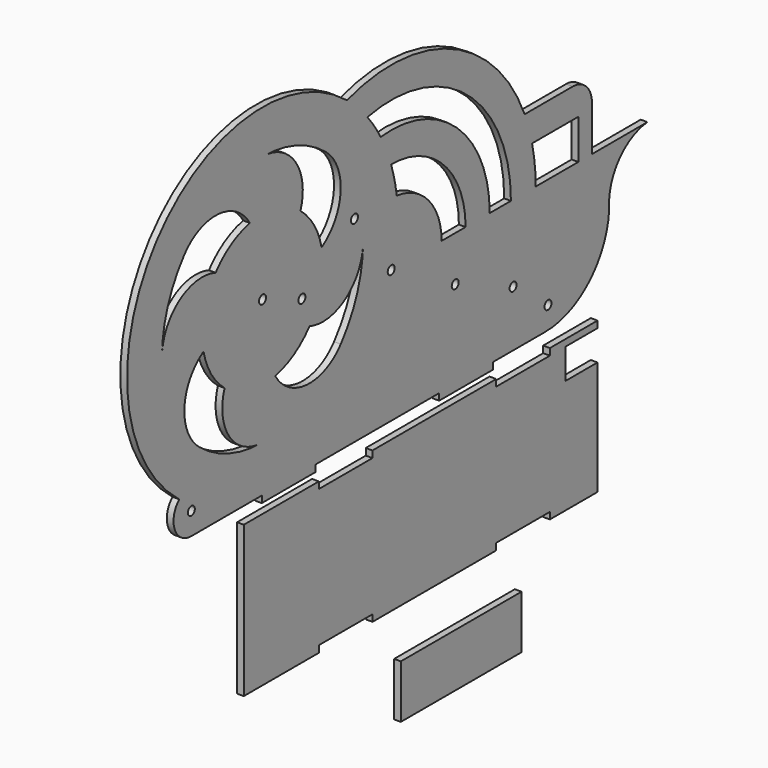
from build123d import *

# Parameters (mm, degrees)
F0_R     = 1.651
F0_W     = 25.4
F0_H     = 2.54
F1_DEPTH = 2.54
F3_DEPTH = 2.54
F2_W     = 57.15
F2_H     = 20.1916538


# Not quite as in the source:
# - a feature names something its author has since deleted; it is built from what else it names


with BuildPart() as f1:
    # F0 (on Right) → F1 (new body)
    with BuildSketch(Plane.YZ):
        with BuildLine():
            Line((-110.3395098078, -68.216781003), (-77.0102134189, -68.216781003))
            Line((-77.0102134189, -68.216781003), (-51.6102134189, -68.216781003))
            Line((-51.6102134189, -68.216781003), (6.9758426398, -68.216781003))
            Line((6.9758426398, -68.216781003), (32.3758426398, -68.216781003))
            Line((32.3758426398, -68.216781003), (57.100551478, -68.216781003))
            ThreePointArc((57.100551478, -68.216781003), (79.1760571871, -58.7450905637), (87.4551682283, -36.1952082478))
            ThreePointArc((87.4551682283, -36.1952082478), (93.1827609105, -23.7752479136), (105.5495773538, -17.933794011))
            Line((105.5495773538, -17.933794011), (79.3032324412, -17.933794011))
            Line((79.3032324412, -17.933794011), (79.3032324412, -0.7903648026))
            ThreePointArc((79.3032324412, -0.7903648026), (76.6409185109, 5.6370295953), (70.2135241129, 8.2993435257))
            Line((70.2135241129, 8.2993435257), (47.4198818769, 8.2993435257))
            ThreePointArc((47.4198818769, 8.2993435257), (12.9543250307, 44.1398405436), (-36.6774012974, 47.1577167678))
            ThreePointArc((-36.6774012974, 47.1577167678), (-127.0218705021, 36.6937065388), (-116.0831372229, -53.5945138457))
            ThreePointArc((-116.0831372229, -53.5945138457), (-118.1944438098, -62.8630173745), (-110.3395098078, -68.216781003))
        make_face()
        with Locations((-110.3395098078, -59.7775988281)):
            Circle(F0_R, mode=Mode.SUBTRACT)
        with BuildLine():
            ThreePointArc((-106.5792463676, -40.0513765479), (-113.6163335987, -24.0126518115), (-104.5836338962, -9.0069321035))
            ThreePointArc((-104.5836338962, -9.0069321035), (-100.986725964, -17.9768034164), (-94.6055715395, -25.2347098813))
            ThreePointArc((-94.6055715395, -25.2347098813), (-92.199319164, -42.5832325093), (-76.6450592973, -50.6347098813))
            ThreePointArc((-76.6450592973, -50.6347098813), (-92.5200592973, -47.9109904866), (-106.5792463676, -40.0513765479))
        make_face(mode=Mode.SUBTRACT)
        with BuildLine():
            ThreePointArc((-70.6478370751, -30.9482844801), (-61.6779657622, -27.3513765479), (-54.4200592973, -20.9702221234))
            ThreePointArc((-54.4200592973, -20.9702221234), (-37.0715366693, -18.5639697479), (-29.0200592973, -3.0097098813))
            ThreePointArc((-29.0200592973, -3.0097098813), (-31.743778692, -18.8847098813), (-39.6033926307, -32.9438969515))
            ThreePointArc((-39.6033926307, -32.9438969515), (-55.6421173671, -39.9809841827), (-70.6478370751, -30.9482844801))
        make_face(mode=Mode.SUBTRACT)
        with Locations((-57.9914643632, -10.3356258236)):
            Circle(F0_R, mode=Mode.SUBTRACT)
        with Locations((41.94092891, -46.9549127524)):
            Circle(F0_R, mode=Mode.SUBTRACT)
        with Locations((58.4825998644, -59.7775988281)):
            Circle(F0_R, mode=Mode.SUBTRACT)
        with Locations((14.561701, -35.0126066428)):
            Circle(F0_R, mode=Mode.SUBTRACT)
        with Locations((-15.7277009394, -17.933794011)):
            Circle(F0_R, mode=Mode.SUBTRACT)
        with BuildLine():
            Line((72.8437239482, -17.933794011), (52.6520820419, -17.933794011))
            ThreePointArc((52.6520820419, -17.933794011), (52.2295051274, -10.343480173), (50.9669973093, -2.8469803618))
            Line((50.9669973093, -2.8469803618), (72.8437239482, -2.8469803618))
            Line((72.8437239482, -2.8469803618), (72.8437239482, -17.933794011))
        make_face(mode=Mode.SUBTRACT)
        with BuildLine():
            ThreePointArc((-124.2700592973, -3.0097098813), (-121.5463399027, 12.8652901187), (-113.686725964, 26.924477189))
            ThreePointArc((-113.686725964, 26.924477189), (-97.6480012275, 33.9615644202), (-82.6422815195, 24.9288647176))
            ThreePointArc((-82.6422815195, 24.9288647176), (-91.6121528324, 21.3319567854), (-98.8700592973, 14.9508023609))
            ThreePointArc((-98.8700592973, 14.9508023609), (-116.2185819254, 12.5445499854), (-124.2700592973, -3.0097098813))
        make_face(mode=Mode.SUBTRACT)
        with Locations((-76.6450592973, -3.0097098813)):
            Circle(F0_R, mode=Mode.SUBTRACT)
        with Locations((-33.1285902436, 6.2196841001)):
            Circle(F0_R, mode=Mode.SUBTRACT)
        with BuildLine():
            ThreePointArc((-46.7108722271, 34.0319567854), (-39.6737849959, 17.993232049), (-48.7064846984, 2.987512341))
            ThreePointArc((-48.7064846984, 2.987512341), (-52.3033926307, 11.9573836539), (-58.6845470552, 19.2152901187))
            ThreePointArc((-58.6845470552, 19.2152901187), (-61.0907994306, 36.5638127468), (-76.6450592973, 44.6152901187))
            ThreePointArc((-76.6450592973, 44.6152901187), (-60.7700592973, 41.8915707241), (-46.7108722271, 34.0319567854))
        make_face(mode=Mode.SUBTRACT)
        with BuildLine():
            ThreePointArc((8.1256330932, -17.933794011), (2.0413714041, -2.0202270784), (-13.1075925996, 5.7752037906))
            ThreePointArc((-13.1075925996, 5.7752037906), (-14.1849392561, 11.581992796), (-15.7918139924, 17.2650754062))
            ThreePointArc((-15.7918139924, 17.2650754062), (9.1390218846, 6.9782636063), (19.4712268672, -17.933794011))
            Line((19.4712268672, -17.933794011), (8.1256330932, -17.933794011))
        make_face(mode=Mode.SUBTRACT)
        with BuildLine():
            ThreePointArc((-26.9908731892, 37.5938144058), (20.1332877639, 25.9314979047), (40.9306995465, -17.933794011))
            Line((40.9306995465, -17.933794011), (30.8992126275, -17.933794011))
            ThreePointArc((30.8992126275, -17.933794011), (15.4225371964, 16.7610432542), (-20.7332734529, 28.4236575215))
            ThreePointArc((-20.7332734529, 28.4236575215), (-23.6633025042, 33.1443746694), (-26.9908731892, 37.5938144058))
        make_face(mode=Mode.SUBTRACT)
        with Locations((-64.3102134189, -69.486781003)):
            Rectangle(F0_W, F0_H)
        with Locations((19.6758426398, -69.486781003)):
            Rectangle(F0_W, F0_H)
    extrude(amount=F1_DEPTH)


with BuildPart() as f3:
    # F2 (on Right) → F3 (new body)
    with BuildSketch(Plane.YZ):
        Polygon((-50.0091612339, -74.4957265361), (-85.5189124058, -74.4957265361), (-85.5189124058, -131.6457265361), (-50.0091612339, -131.6457265361), (-50.0091612339, -129.1057265361), (-24.6091612339, -129.1057265361), (-24.6091612339, -131.6457265361), (33.9769039661, -131.6457265361), (33.9769039661, -129.1057265361), (59.3769039661, -129.1057265361), (59.3769039661, -131.6457265361), (81.9211387942, -131.6457265361), (81.9211387942, -88.4657265361), (66.6811387942, -88.4657265361), (66.6811387942, -77.0357265361), (81.9211387942, -77.0357265361), (81.9211387942, -74.4957265361), (59.3769039661, -74.4957265361), (59.3769039661, -77.0357265361), (33.9769039661, -77.0357265361), (33.9769039661, -74.4957265361), (-24.6091612339, -74.4957265361), (-24.6091612339, -77.0357265361), (-50.0091612339, -77.0357265361), align=None)
    extrude(amount=F3_DEPTH)


with BuildPart() as f3b:
    # F2 (on Right) → F3, piece 2 (new body)
    with BuildSketch(Plane.YZ):
        with Locations((17.3918033212, -160.3580791593)):
            Rectangle(F2_W, F2_H)
    extrude(amount=F3_DEPTH)


solid = Compound([f1.part, f3.part, f3b.part])
